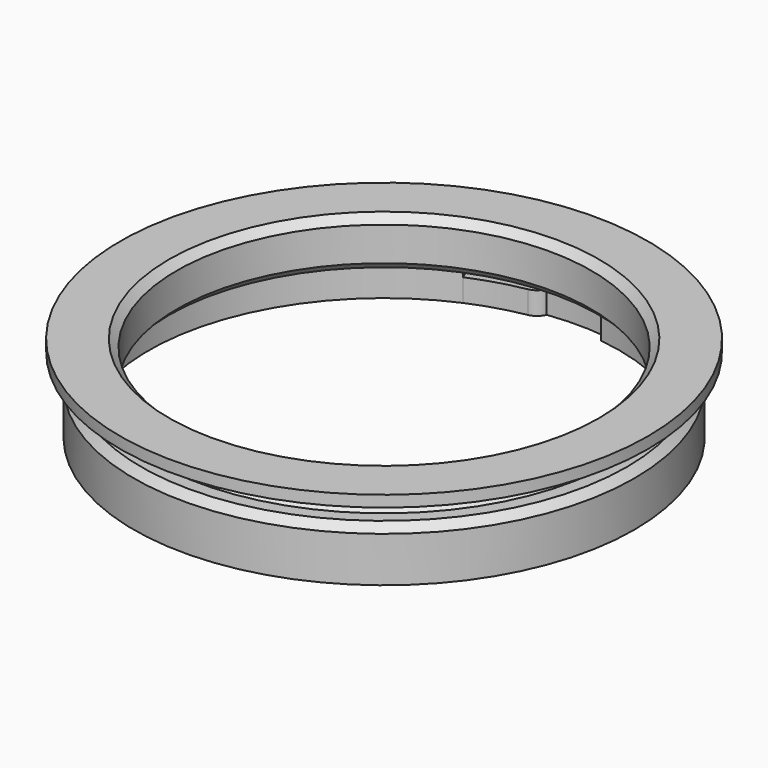
from build123d import *
from build123d import SkipClean  # not in build123d's __all__

# Parameters (mm, degrees)
F0_W        = 2
F0_H        = 2
F0_H_2      = 3
F2_SIZE     = 1
F4_DEPTH    = 5
F5_DEPTH    = 3
F6_T4_DEPTH = 10.6380386618
F6_T6_DEPTH = 6.8190193309
F6_T8_DEPTH = 6.8190193309


# Not quite as in the source:
# - a fillet or chamfer that OpenCascade refuses, or shapes differently, is made with other operations: its cross-section is extruded or revolved along the edge and cut away or added


with BuildPart() as f1:
    # F0 (on Front) → F1 (revolve)
    with BuildSketch(Plane.XZ):
        Polygon((33.2, -3.5), (33.2, 3.5), (29.5090141887, 3.5), (29.5090141887, 1.5), (31.2, 1.5), (31.2, -3.5), align=None)
        with Locations((28.5090141887, 2.5)):
            Rectangle(F0_W, F0_H)
        with Locations((28.5090141887, 5)):
            Rectangle(F0_W, F0_H_2)
        Polygon((27.5090141887, 6.5), (29.5090141887, 6.5), (35, 6.5), (35, 8), (27.5090141887, 8), align=None)
    revolve(axis=Axis((0, 0, 0.081283506), (0, 0, -1)))

    # F2
    f2_edges = [f1.edges().sort_by_distance(p)[0] for p in [
        (-33.2, 0, 3.5),
        (-27.509014, 0, 1.5),
        (-29.509014, 0, 3.5),
        (-27.509014, 0, 8),
    ]]
    chamfer(f2_edges, length=F2_SIZE)

    # F3 (on face) → F4 (cut, through all)
    with BuildSketch(Plane(origin=(0, 0, -3.5), x_dir=(1, 0, 0), z_dir=(0, 0, -1))):
        with BuildLine():
            ThreePointArc((-4, -31.9505868491), (0, -32.2), (4, -31.9505868491))
            Line((4, -31.9505868491), (4, -30.9425273693))
            ThreePointArc((4, -30.9425273693), (0, -31.2), (-4, -30.9425273693))
            Line((-4, -30.9425273693), (-4, -31.9505868491))
        make_face()
        with BuildLine():
            ThreePointArc((-12.8274571452, -29.5346634176), (-8.5, -31.0578492494), (-4, -31.9505868491))
            Line((-4, -31.9505868491), (-4, -30.9425273693))
            ThreePointArc((-4, -30.9425273693), (-8.2963998779, -30.0767310236), (-12.4290889109, -28.6174378456))
            Line((-12.4290889109, -28.6174378456), (-12.8274571452, -29.5346634176))
        make_face()
        with BuildLine():
            ThreePointArc((-25.6700198771, 19.4393950397), (-27.8860180019, 16.1), (-29.6700198771, 12.5111918094))
            Line((-29.6700198771, 12.5111918094), (-28.7970147591, 12.0071620695))
            ThreePointArc((-28.7970147591, 12.0071620695), (-27.0199925981, 15.6), (-24.7970147591, 18.9353652998))
            Line((-24.7970147591, 18.9353652998), (-25.6700198771, 19.4393950397))
        make_face()
        with BuildLine():
            Line((-18.5688837101, 25.0726256655), (-19.1640402392, 25.8762354625))
            ThreePointArc((-19.1640402392, 25.8762354625), (-22.6468864369, 22.8901405569), (-25.6700198771, 19.4393950397))
            Line((-25.6700198771, 19.4393950397), (-24.7970147591, 18.9353652998))
            ThreePointArc((-24.7970147591, 18.9353652998), (-21.8990131903, 22.223258566), (-18.5688837101, 25.0726256655))
        make_face()
        with BuildLine():
            Line((30.9979726209, 3.5448121801), (31.9914973844, 3.6584279551))
            ThreePointArc((31.9914973844, 3.6584279551), (31.1468864369, 8.1677086925), (29.6700198771, 12.5111918094))
            Line((29.6700198771, 12.5111918094), (28.7970147591, 12.0071620695))
            ThreePointArc((28.7970147591, 12.0071620695), (30.1954130682, 7.8534724576), (30.9979726209, 3.5448121801))
        make_face()
        with BuildLine():
            Line((28.7970147591, 12.0071620695), (29.6700198771, 12.5111918094))
            ThreePointArc((29.6700198771, 12.5111918094), (27.8860180019, 16.1), (25.6700198771, 19.4393950397))
            Line((25.6700198771, 19.4393950397), (24.7970147591, 18.9353652998))
            ThreePointArc((24.7970147591, 18.9353652998), (27.0199925981, 15.6), (28.7970147591, 12.0071620695))
        make_face()
    extrude(amount=-F4_DEPTH, mode=Mode.SUBTRACT)

    # F3 (on face) → F5 (join)
    with BuildSketch(Plane(origin=(0, 0, -3.5), x_dir=(1, 0, 0), z_dir=(0, 0, -1))):
        with BuildLine():
            ThreePointArc((4, -31.9505868491), (24.1416652284, -21.3077450707), (32.2, 0))
            ThreePointArc((32.2, 0), (32.1478320869, 1.8321823356), (31.9914973844, 3.6584279551))
            Line((31.9914973844, 3.6584279551), (30.9979726209, 3.5448121801))
            ThreePointArc((30.9979726209, 3.5448121801), (31.1494522084, 1.775282263), (31.2, 0))
            ThreePointArc((31.2, 0), (23.4333096254, -20.5990291033), (4, -30.9425273693))
            Line((4, -30.9425273693), (4, -31.9505868491))
        make_face()
        with BuildLine():
            Line((30.9979726209, 3.5448121801), (31.9914973844, 3.6584279551))
            ThreePointArc((31.9914973844, 3.6584279551), (31.1468864369, 8.1677086925), (29.6700198771, 12.5111918094))
            Line((29.6700198771, 12.5111918094), (28.7970147591, 12.0071620695))
            ThreePointArc((28.7970147591, 12.0071620695), (30.1954130682, 7.8534724576), (30.9979726209, 3.5448121801))
        make_face()
        with BuildLine():
            ThreePointArc((-12.8274571452, -29.5346634176), (-8.5, -31.0578492494), (-4, -31.9505868491))
            Line((-4, -31.9505868491), (-4, -30.9425273693))
            ThreePointArc((-4, -30.9425273693), (-8.2963998779, -30.0767310236), (-12.4290889109, -28.6174378456))
            Line((-12.4290889109, -28.6174378456), (-12.8274571452, -29.5346634176))
        make_face()
        with BuildLine():
            Line((-18.5688837101, 25.0726256655), (-19.1640402392, 25.8762354625))
            ThreePointArc((-19.1640402392, 25.8762354625), (-22.6468864369, 22.8901405569), (-25.6700198771, 19.4393950397))
            Line((-25.6700198771, 19.4393950397), (-24.7970147591, 18.9353652998))
            ThreePointArc((-24.7970147591, 18.9353652998), (-21.8990131903, 22.223258566), (-18.5688837101, 25.0726256655))
        make_face()
    with SkipClean():  # cleaning this boolean's faces spoils the solid; the shape is the same uncleaned
        extrude(amount=-F5_DEPTH)

    # F6: fillet of radius 2 on 3 edges, made by hand


with BuildPart() as f6_tool2:
    # F6_s3 → F6_t4 (new body)
    with BuildSketch(Plane.XY.offset(-7.3190193309)):
        with BuildLine():
            ThreePointArc((-4, 31.9505868491), (-4.5929852552, 31.1331579467), (-5.5097528505, 30.7096503322))
            ThreePointArc((-5.5097528505, 30.7096503322), (-4.7563018983, 30.8353302601), (-4, 30.9425273693))
            Line((-4, 30.9425273693), (-4, 31.9505868491))
        make_face()
    extrude(amount=F6_T4_DEPTH)

    split(bisect_by=Plane.XY.offset(1.5), keep=Keep.BOTTOM)


with BuildPart() as f1_1:
    add(f1.part, clean=False)

    # F6_t1: cut F6_tool2
    add(f6_tool2.part, mode=Mode.SUBTRACT)

    # F6_s7 → F6_t6 (cut)
    with BuildSketch(Plane.XY.offset(-7.3190193309)):
        with BuildLine():
            ThreePointArc((-25.6700198771, -19.4393950397), (-24.6656130543, -19.5442208835), (-23.8404609038, -20.1264111032))
            ThreePointArc((-23.8404609038, -20.1264111032), (-24.3260283902, -19.5367434021), (-24.7970147591, -18.9353652998))
            Line((-24.7970147591, -18.9353652998), (-25.6700198771, -19.4393950397))
        make_face()
    extrude(amount=F6_T6_DEPTH, mode=Mode.SUBTRACT)

    # F6_s9 → F6_t8 (cut)
    with BuildSketch(Plane.XY.offset(-7.3190193309)):
        with BuildLine():
            ThreePointArc((29.6700198771, -12.5111918094), (29.2585983094, -11.5889370631), (29.3502137543, -10.583239229))
            ThreePointArc((29.3502137543, -10.583239229), (29.0823302885, -11.2985868581), (28.7970147591, -12.0071620695))
            Line((28.7970147591, -12.0071620695), (29.6700198771, -12.5111918094))
        make_face()
    extrude(amount=F6_T8_DEPTH, mode=Mode.SUBTRACT)


solid = f1_1.part
